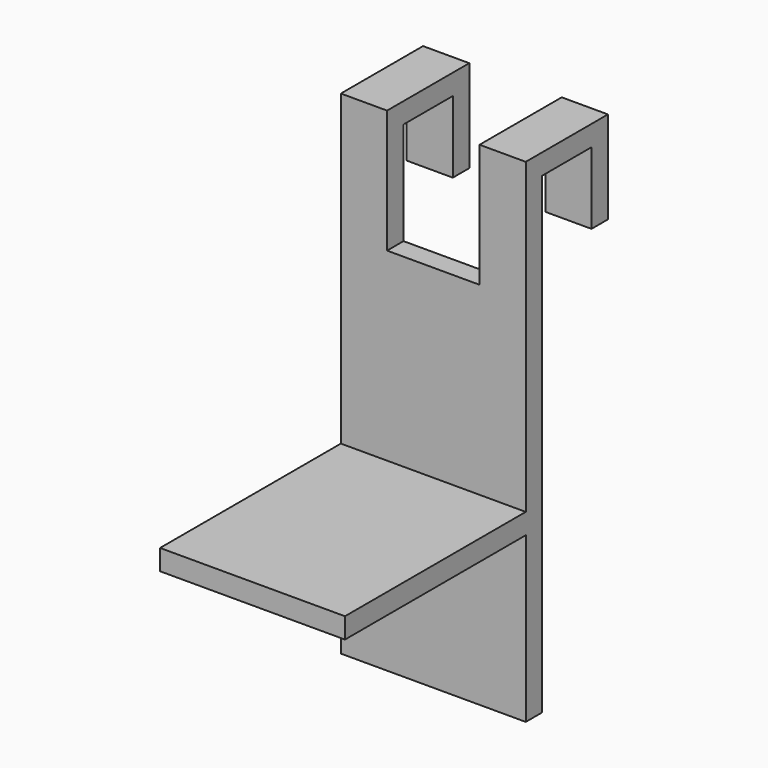
from build123d import *

# Parameters (mm, degrees)
F1_DEPTH = 25.4
F2_W     = 57.15
F2_H     = 25.4
F3_DEPTH = 76.2
F4_W     = 57.15
F4_H     = 25.4
F5_DEPTH = 114.3
F6_W     = 57.15
F6_H     = 25.4
F7_DEPTH = 114.3
F8_W     = 228.6
F8_H     = 25.4
F9_DEPTH = 279.4


with BuildPart() as f1:
    # F0 (on Front) → F1 (new body)
    with BuildSketch(Plane.XZ):
        Polygon((-171.4900614394, 291.4170305759), (-228.6400614394, 291.4170305759), (-228.6400614394, -318.1829694241), (-0.0400614394, -318.1829694241), (-0.0400614394, 291.4170305759), (-57.1900614394, 291.4170305759), (-57.1900614394, 139.0170305759), (-171.4900614394, 139.0170305759), align=None)
    extrude(amount=F1_DEPTH)

    # F2 (on face) → F3 (join)
    with BuildSketch(Plane(origin=(0, 0, 0), x_dir=(-1, 0, 0), z_dir=(0, 1, 0))):
        with Locations((28.6150614394, 278.7170305759)):
            Rectangle(F2_W, F2_H)
        with Locations((200.0650614394, 278.7170305759)):
            Rectangle(F2_W, F2_H)
    extrude(amount=F3_DEPTH)

    # F4 (on face) → F5 (join)
    with BuildSketch(Plane.XY.offset(291.4170305759)):
        with Locations((-28.6150614394, 88.9)):
            Rectangle(F4_W, F4_H)
    extrude(amount=-F5_DEPTH)

    # F6 (on face) → F7 (join)
    with BuildSketch(Plane.XY.offset(291.4170305759)):
        with Locations((-200.0650614394, 88.9)):
            Rectangle(F6_W, F6_H)
    extrude(amount=-F7_DEPTH)

    # F8 (on face) → F9 (join)
    with BuildSketch(Plane.XZ.offset(25.4)):
        with Locations((-114.3400614394, -102.2829694241)):
            Rectangle(F8_W, F8_H)
    extrude(amount=F9_DEPTH)


solid = f1.part
